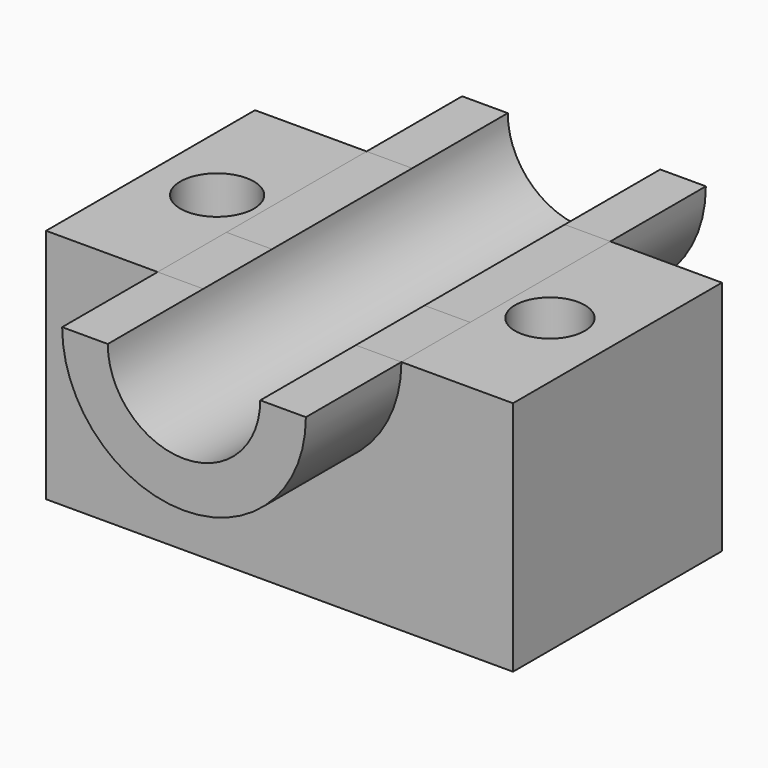
from build123d import *

# Parameters (mm, degrees)
F1_DEPTH = 73.914
F2_DEPTH = 38.608
F3_DEPTH = 25.4
F4_DEPTH = 87.123
F5_R     = 10.8850211106
F5_R_2   = 10.3170822269
F6_DEPTH = 69.8849575052


with BuildPart() as f1:
    # F0 (on Front) → F1 (new body, symmetric)
    with BuildSketch(Plane.XZ):
        with BuildLine():
            ThreePointArc((-36.0318907806, 34.9419787526), (0, -1.089912028), (36.0318907806, 34.9419787526))
            Line((36.0318907806, 34.9419787526), (22.5412292513, 34.9419787526))
            ThreePointArc((22.5412292513, 34.9419787526), (0, 12.4007495013), (-22.5412292513, 34.9419787526))
            Line((-22.5412292513, 34.9419787526), (-36.0318907806, 34.9419787526))
        make_face()
    extrude(amount=F1_DEPTH, both=True)

    # F0 (on Front) → F2 (join, symmetric)
    with BuildSketch(Plane.XZ):
        with BuildLine():
            Line((69.0282359719, -34.9419787526), (69.0282359719, 34.9419787526))
            Line((69.0282359719, 34.9419787526), (36.0318907806, 34.9419787526))
            ThreePointArc((36.0318907806, 34.9419787526), (0, -1.089912028), (-36.0318907806, 34.9419787526))
            Line((-36.0318907806, 34.9419787526), (-69.0282359719, 34.9419787526))
            Line((-69.0282359719, 34.9419787526), (-69.0282359719, -34.9419787526))
            Line((-69.0282359719, -34.9419787526), (69.0282359719, -34.9419787526))
        make_face()
        with BuildLine():
            ThreePointArc((-36.0318907806, 34.9419787526), (0, -1.089912028), (36.0318907806, 34.9419787526))
            Line((36.0318907806, 34.9419787526), (22.5412292513, 34.9419787526))
            ThreePointArc((22.5412292513, 34.9419787526), (0, 12.4007495013), (-22.5412292513, 34.9419787526))
            Line((-22.5412292513, 34.9419787526), (-36.0318907806, 34.9419787526))
        make_face()
        with BuildLine():
            Line((22.5412292513, 34.9419787526), (36.0318907806, 34.9419787526))
            ThreePointArc((36.0318907806, 34.9419787526), (0, 70.9738695332), (-36.0318907806, 34.9419787526))
            Line((-36.0318907806, 34.9419787526), (-22.5412292513, 34.9419787526))
            ThreePointArc((-22.5412292513, 34.9419787526), (0, 57.4832080039), (22.5412292513, 34.9419787526))
        make_face()
    extrude(amount=F2_DEPTH, both=True)

    # F3 (cut): a face of the model
    f3_faces = [f1.faces().sort_by_distance(p)[0] for p in [
        (29.286560016, -38.608, 35.747676324),
    ]]
    extrude(f3_faces, amount=-F3_DEPTH, mode=Mode.SUBTRACT)

    # F4 (cut, through all): a face of the model
    f4_faces = [f1.faces().sort_by_distance(p)[0] for p in [
        (29.286560016, -13.208, 35.747676324),
    ]]
    extrude(f4_faces, amount=-F4_DEPTH, mode=Mode.SUBTRACT)

    # F5 (on face) → F6 (cut, through all)
    with BuildSketch(Plane.XY.offset(34.9419787526)):
        with Locations((-49.3466295302, 0)):
            Circle(F5_R)
        with Locations((49.0613915026, 0)):
            Circle(F5_R_2)
    extrude(amount=-F6_DEPTH, mode=Mode.SUBTRACT)


solid = f1.part
